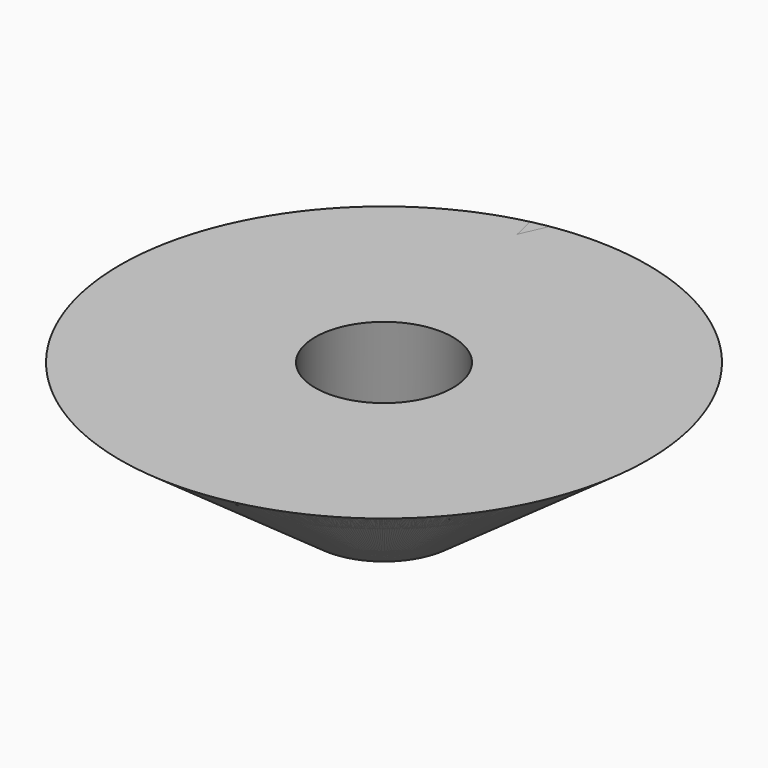
from build123d import *

# Parameters (mm, degrees)
F2_DEPTH = 30
F4_DEPTH = 25
F5_COUNT = 28


with BuildPart() as f1:
    # F0 (on Front) → F1 (revolve)
    with BuildSketch(Plane.XZ):
        Polygon((-51.0810799897, 36.5230441093), (0, 0), (18.0286169052, 0), (18.0286169052, 10.1701514795), (0, 10.1701514795), (0, 36.5230441093), align=None)
    revolve(axis=Axis((18.0286169052, 0, 5.0850757398), (0, 0, -1)))

    # F2 (cut): a face of the model
    f2_faces = [f1.faces().sort_by_distance(p)[0] for p in [
        (18.0286169052, 0, 10.1701514795),
    ]]
    extrude(f2_faces, amount=-F2_DEPTH, mode=Mode.SUBTRACT)

    # F3 (on face) → F4 (cut)
    with BuildSketch(Plane.XY.offset(36.5230441093)):
        with BuildLine():
            ThreePointArc((22.3380177721, 68.9752076407), (20.0890180785, 69.0789761933), (17.8378317505, 69.1094335524))
            Line((17.8378317505, 69.1094335524), (17.8378317505, 62.9749596119))
            Line((17.8378317505, 62.9749596119), (22.3380177721, 68.9752076407))
        make_face()
    extrude(amount=-F4_DEPTH, mode=Mode.SUBTRACT)


with BuildPart() as f5_1:
    # F5: instance of F1
    add(f1.part.rotate(Axis((18.0286169052, 0, 36.5230441093), (0, 0, -1)), 1 * 360 / F5_COUNT))


with BuildPart() as f5_2:
    # F5: instance of F1
    add(f1.part.rotate(Axis((18.0286169052, 0, 36.5230441093), (0, 0, -1)), 2 * 360 / F5_COUNT))


with BuildPart() as f5_3:
    # F5: instance of F1
    add(f1.part.rotate(Axis((18.0286169052, 0, 36.5230441093), (0, 0, -1)), 3 * 360 / F5_COUNT))


with BuildPart() as f5_4:
    # F5: instance of F1
    add(f1.part.rotate(Axis((18.0286169052, 0, 36.5230441093), (0, 0, -1)), 4 * 360 / F5_COUNT))


with BuildPart() as f5_5:
    # F5: instance of F1
    add(f1.part.rotate(Axis((18.0286169052, 0, 36.5230441093), (0, 0, -1)), 5 * 360 / F5_COUNT))


with BuildPart() as f5_6:
    # F5: instance of F1
    add(f1.part.rotate(Axis((18.0286169052, 0, 36.5230441093), (0, 0, -1)), 6 * 360 / F5_COUNT))


with BuildPart() as f5_7:
    # F5: instance of F1
    add(f1.part.rotate(Axis((18.0286169052, 0, 36.5230441093), (0, 0, -1)), 7 * 360 / F5_COUNT))


with BuildPart() as f5_8:
    # F5: instance of F1
    add(f1.part.rotate(Axis((18.0286169052, 0, 36.5230441093), (0, 0, -1)), 8 * 360 / F5_COUNT))


with BuildPart() as f5_9:
    # F5: instance of F1
    add(f1.part.rotate(Axis((18.0286169052, 0, 36.5230441093), (0, 0, -1)), 9 * 360 / F5_COUNT))


with BuildPart() as f5_10:
    # F5: instance of F1
    add(f1.part.rotate(Axis((18.0286169052, 0, 36.5230441093), (0, 0, -1)), 10 * 360 / F5_COUNT))


with BuildPart() as f5_11:
    # F5: instance of F1
    add(f1.part.rotate(Axis((18.0286169052, 0, 36.5230441093), (0, 0, -1)), 11 * 360 / F5_COUNT))


with BuildPart() as f5_12:
    # F5: instance of F1
    add(f1.part.rotate(Axis((18.0286169052, 0, 36.5230441093), (0, 0, -1)), 12 * 360 / F5_COUNT))


with BuildPart() as f5_13:
    # F5: instance of F1
    add(f1.part.rotate(Axis((18.0286169052, 0, 36.5230441093), (0, 0, -1)), 13 * 360 / F5_COUNT))


with BuildPart() as f5_14:
    # F5: instance of F1
    add(f1.part.rotate(Axis((18.0286169052, 0, 36.5230441093), (0, 0, -1)), 14 * 360 / F5_COUNT))


with BuildPart() as f5_15:
    # F5: instance of F1
    add(f1.part.rotate(Axis((18.0286169052, 0, 36.5230441093), (0, 0, -1)), 15 * 360 / F5_COUNT))


with BuildPart() as f5_16:
    # F5: instance of F1
    add(f1.part.rotate(Axis((18.0286169052, 0, 36.5230441093), (0, 0, -1)), 16 * 360 / F5_COUNT))


with BuildPart() as f5_17:
    # F5: instance of F1
    add(f1.part.rotate(Axis((18.0286169052, 0, 36.5230441093), (0, 0, -1)), 17 * 360 / F5_COUNT))


with BuildPart() as f5_18:
    # F5: instance of F1
    add(f1.part.rotate(Axis((18.0286169052, 0, 36.5230441093), (0, 0, -1)), 18 * 360 / F5_COUNT))


with BuildPart() as f5_19:
    # F5: instance of F1
    add(f1.part.rotate(Axis((18.0286169052, 0, 36.5230441093), (0, 0, -1)), 19 * 360 / F5_COUNT))


with BuildPart() as f5_20:
    # F5: instance of F1
    add(f1.part.rotate(Axis((18.0286169052, 0, 36.5230441093), (0, 0, -1)), 20 * 360 / F5_COUNT))


with BuildPart() as f5_21:
    # F5: instance of F1
    add(f1.part.rotate(Axis((18.0286169052, 0, 36.5230441093), (0, 0, -1)), 21 * 360 / F5_COUNT))


with BuildPart() as f5_22:
    # F5: instance of F1
    add(f1.part.rotate(Axis((18.0286169052, 0, 36.5230441093), (0, 0, -1)), 22 * 360 / F5_COUNT))


with BuildPart() as f5_23:
    # F5: instance of F1
    add(f1.part.rotate(Axis((18.0286169052, 0, 36.5230441093), (0, 0, -1)), 23 * 360 / F5_COUNT))


with BuildPart() as f5_24:
    # F5: instance of F1
    add(f1.part.rotate(Axis((18.0286169052, 0, 36.5230441093), (0, 0, -1)), 24 * 360 / F5_COUNT))


with BuildPart() as f5_25:
    # F5: instance of F1
    add(f1.part.rotate(Axis((18.0286169052, 0, 36.5230441093), (0, 0, -1)), 25 * 360 / F5_COUNT))


with BuildPart() as f5_26:
    # F5: instance of F1
    add(f1.part.rotate(Axis((18.0286169052, 0, 36.5230441093), (0, 0, -1)), 26 * 360 / F5_COUNT))


with BuildPart() as f5_27:
    # F5: instance of F1
    add(f1.part.rotate(Axis((18.0286169052, 0, 36.5230441093), (0, 0, -1)), 27 * 360 / F5_COUNT))


solid = Compound([f1.part, f5_1.part, f5_2.part, f5_3.part, f5_4.part, f5_5.part, f5_6.part, f5_7.part, f5_8.part, f5_9.part, f5_10.part, f5_11.part, f5_12.part, f5_13.part, f5_14.part, f5_15.part, f5_16.part, f5_17.part, f5_18.part, f5_19.part, f5_20.part, f5_21.part, f5_22.part, f5_23.part, f5_24.part, f5_25.part, f5_26.part, f5_27.part])
